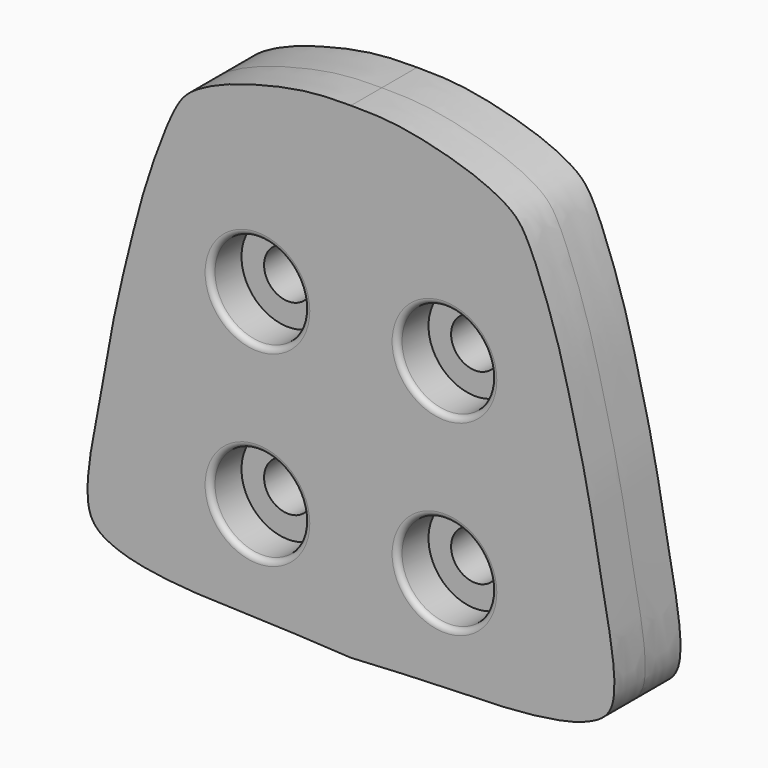
from build123d import *

# Parameters (mm, degrees)
F0_R     = 2.125
F0_R_2   = 1.1
F1_DEPTH = 2
F2_DEPTH = 3.75
F3_R     = 0.25


# Not quite as in the source:
# - a feature of the source that left no trace in its solid (it failed there, or was rolled back) is left out


with BuildPart() as f1:
    # F0 (on Front) → F1 (new body)
    with BuildSketch(Plane.XZ):
        with BuildLine():
            Line((-11.2853205, -2.761329), (-11.8082743138, -5.6065687805))
            add(Edge.make_bspline(
                [(-11.8082743138, -5.6065687805), (-11.9499793699, -6.5386188687), (-12.1160849764, -8.2018960588), (-10.9538603761, -9.0113788314), (-9.4881850802, -9.4440964683), (-7.3079859676, -9.6905458476), (-5.1732434914, -9.7425713575), (-2.6347207257, -9.8273186305), (-0.8783558838, -9.9244436474), (0, -9.973105)],
                knots=[0.6030919147, 0.6030919147, 0.6030919147, 0.6030919147, 0.6656030044, 0.7084220489, 0.7568845459, 0.8150973045, 0.873110022, 0.9357637082, 1, 1, 1, 1], degree=3))
            add(Edge.make_bspline(
                [(0, 12.0851723477), (0.9551344788, 12.0937472566), (2.3485794737, 12.0150050235), (4.6831228194, 11.4504344151), (6.1961787746, 10.9108739557), (7.3603958573, 10.268692138), (8.0707440931, 9.4041166376), (9.2414301503, 6.2609292886), (9.8616147158, 3.9450852254), (10.8191617953, 0.0558623263), (11.2532218847, -2.7347737553), (11.8442674277, -5.4800858922), (12.1160849764, -8.2018960588), (10.9538603761, -9.0113788314), (9.4881850802, -9.4440964683), (7.3079859676, -9.6905458476), (5.1732434914, -9.7425713575), (2.6347207257, -9.8273186305), (0.8783558838, -9.9244436474), (0, -9.973105)],
                knots=[0, 0, 0, 0, 0.061518357, 0.1215232323, 0.1719600852, 0.2155897239, 0.256825018, 0.3273753313, 0.3912499287, 0.4690247596, 0.5360583372, 0.6030919147, 0.6656030044, 0.7084220489, 0.7568845459, 0.8150973045, 0.873110022, 0.9357637082, 1, 1, 1, 1], degree=3))
            add(Edge.make_bspline(
                [(0, 12.0851723477), (-0.9551344788, 12.0937472566), (-2.3485794737, 12.0150050235), (-4.6831228194, 11.4504344151), (-6.1961787746, 10.9108739557), (-7.3603958573, 10.268692138), (-8.0707440931, 9.4041166376), (-9.2414301503, 6.2609292886), (-9.8616147158, 3.9450852254), (-10.5115765842, 1.3051663784), (-10.7623666862, 0.0839107805)],
                knots=[0, 0, 0, 0, 0.061518357, 0.1215232323, 0.1719600852, 0.2155897239, 0.256825018, 0.3273753313, 0.3912499287, 0.4690247596, 0.4690247596, 0.4690247596, 0.4690247596], degree=3))
            Line((-10.7623666862, 0.0839107805), (-11.2398937874, -2.5141754531))
            add(Edge.make_bspline(
                [(-11.2398937874, -2.5141754531), (-11.2548268967, -2.5964389646), (-11.2699414976, -2.6787746124), (-11.2853205, -2.761329)],
                knots=[0.5299744481, 0.5299744481, 0.5299744481, 0.5299744481, 0.5360583372, 0.5360583372, 0.5360583372, 0.5360583372], degree=3))
        make_face()
        with Locations((-4.242641, -5.215746)):
            Circle(F0_R, mode=Mode.SUBTRACT)
        with Locations((4.242641, -5.215746)):
            Circle(F0_R, mode=Mode.SUBTRACT)
        with Locations((-4.242641, 3.269536)):
            Circle(F0_R, mode=Mode.SUBTRACT)
        with Locations((4.242641, 3.269536)):
            Circle(F0_R, mode=Mode.SUBTRACT)
        with Locations((4.242641, 3.269536)):
            Circle(F0_R)
        with Locations((4.242641, 3.269536)):
            Circle(F0_R_2, mode=Mode.SUBTRACT)
        with Locations((4.242641, -5.215746)):
            Circle(F0_R)
        with Locations((4.242641, -5.215746)):
            Circle(F0_R_2, mode=Mode.SUBTRACT)
        with Locations((-4.242641, -5.215746)):
            Circle(F0_R)
        with Locations((-4.242641, -5.215746)):
            Circle(F0_R_2, mode=Mode.SUBTRACT)
        with Locations((-4.242641, 3.269536)):
            Circle(F0_R)
        with Locations((-4.242641, 3.269536)):
            Circle(F0_R_2, mode=Mode.SUBTRACT)
    extrude(amount=F1_DEPTH)

    # F0 (on Front) → F2 (join)
    with BuildSketch(Plane.XZ):
        with BuildLine():
            Line((-11.2853205, -2.761329), (-11.8082743138, -5.6065687805))
            add(Edge.make_bspline(
                [(-11.8082743138, -5.6065687805), (-11.9499793699, -6.5386188687), (-12.1160849764, -8.2018960588), (-10.9538603761, -9.0113788314), (-9.4881850802, -9.4440964683), (-7.3079859676, -9.6905458476), (-5.1732434914, -9.7425713575), (-2.6347207257, -9.8273186305), (-0.8783558838, -9.9244436474), (0, -9.973105)],
                knots=[0.6030919147, 0.6030919147, 0.6030919147, 0.6030919147, 0.6656030044, 0.7084220489, 0.7568845459, 0.8150973045, 0.873110022, 0.9357637082, 1, 1, 1, 1], degree=3))
            add(Edge.make_bspline(
                [(0, 12.0851723477), (0.9551344788, 12.0937472566), (2.3485794737, 12.0150050235), (4.6831228194, 11.4504344151), (6.1961787746, 10.9108739557), (7.3603958573, 10.268692138), (8.0707440931, 9.4041166376), (9.2414301503, 6.2609292886), (9.8616147158, 3.9450852254), (10.8191617953, 0.0558623263), (11.2532218847, -2.7347737553), (11.8442674277, -5.4800858922), (12.1160849764, -8.2018960588), (10.9538603761, -9.0113788314), (9.4881850802, -9.4440964683), (7.3079859676, -9.6905458476), (5.1732434914, -9.7425713575), (2.6347207257, -9.8273186305), (0.8783558838, -9.9244436474), (0, -9.973105)],
                knots=[0, 0, 0, 0, 0.061518357, 0.1215232323, 0.1719600852, 0.2155897239, 0.256825018, 0.3273753313, 0.3912499287, 0.4690247596, 0.5360583372, 0.6030919147, 0.6656030044, 0.7084220489, 0.7568845459, 0.8150973045, 0.873110022, 0.9357637082, 1, 1, 1, 1], degree=3))
            add(Edge.make_bspline(
                [(0, 12.0851723477), (-0.9551344788, 12.0937472566), (-2.3485794737, 12.0150050235), (-4.6831228194, 11.4504344151), (-6.1961787746, 10.9108739557), (-7.3603958573, 10.268692138), (-8.0707440931, 9.4041166376), (-9.2414301503, 6.2609292886), (-9.8616147158, 3.9450852254), (-10.5115765842, 1.3051663784), (-10.7623666862, 0.0839107805)],
                knots=[0, 0, 0, 0, 0.061518357, 0.1215232323, 0.1719600852, 0.2155897239, 0.256825018, 0.3273753313, 0.3912499287, 0.4690247596, 0.4690247596, 0.4690247596, 0.4690247596], degree=3))
            Line((-10.7623666862, 0.0839107805), (-11.2398937874, -2.5141754531))
            add(Edge.make_bspline(
                [(-11.2398937874, -2.5141754531), (-11.2548268967, -2.5964389646), (-11.2699414976, -2.6787746124), (-11.2853205, -2.761329)],
                knots=[0.5299744481, 0.5299744481, 0.5299744481, 0.5299744481, 0.5360583372, 0.5360583372, 0.5360583372, 0.5360583372], degree=3))
        make_face()
        with Locations((-4.242641, -5.215746)):
            Circle(F0_R, mode=Mode.SUBTRACT)
        with Locations((4.242641, -5.215746)):
            Circle(F0_R, mode=Mode.SUBTRACT)
        with Locations((-4.242641, 3.269536)):
            Circle(F0_R, mode=Mode.SUBTRACT)
        with Locations((4.242641, 3.269536)):
            Circle(F0_R, mode=Mode.SUBTRACT)
    extrude(amount=F2_DEPTH)

    # F3
    f3_edges = [f1.edges().sort_by_distance(p)[0] for p in [
        (-6.367641, -3.75, 3.269536),
        (2.117641, -3.75, 3.269536),
        (2.117641, -3.75, -5.215746),
        (-6.367641, -3.75, -5.215746),
    ]]
    fillet(f3_edges, radius=F3_R)


solid = f1.part
